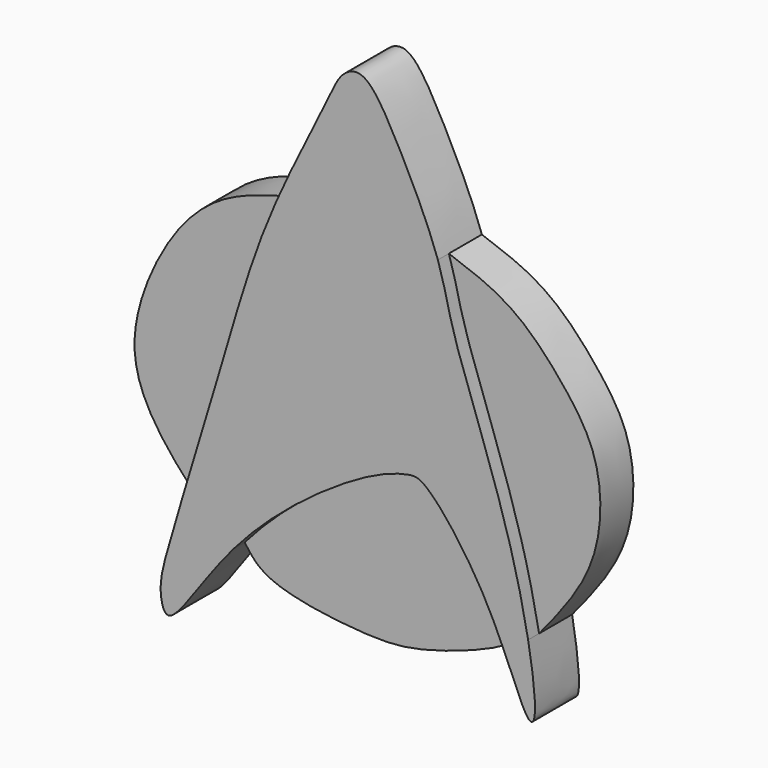
from build123d import *

# Parameters (mm, degrees)
F1_DEPTH = 10.16
F2_DEPTH = 7.62


# Not quite as in the source:
# - a feature names something its author has since deleted; it is built from what else it names


with BuildPart() as f1:
    # F0 (on Front) → F1 (new body)
    with BuildSketch(Plane.XZ):
        with BuildLine():
            add(Edge.make_bspline(
                [(28.992260687, -51.125045095), (28.3542685584, -47.6041133313), (24.5731440192, -30.3142446822), (14.6542496305, -6.5082500378), (13.6472214399, 1.3233310586), (12.3196523637, 5.2555091679)],
                knots=[0.8432322735, 0.8432322735, 0.8432322735, 0.8432322735, 0.8677839764, 0.9518885045, 1, 1, 1, 1], degree=3))
            add(Edge.make_bspline(
                [(12.3196523637, 5.2555091679), (10.61980651, 10.290348239), (4.9500571604, 22.0767618937), (-0.9757985337, 31.9404522882), (-5.7479640246, 30.0120107701), (-8.2004857079, 23.9136843789), (-14.3824154124, 12.2416093831), (-17.6358987441, 4.8334208231)],
                knots=[0, 0, 0, 0, 0.0616029159, 0.1066291224, 0.1322179197, 0.1677258873, 0.2305197427, 0.2305197427, 0.2305197427, 0.2305197427], degree=3))
            add(Edge.make_bspline(
                [(-17.6358987441, 4.8334208231), (-17.9733857287, 4.0649622317), (-22.1836405162, -5.7326263077), (-26.4141695975, -20.9824695343), (-32.763153948, -41.7024504699), (-34.8875297492, -48.7852445916)],
                knots=[0.2305197427, 0.2305197427, 0.2305197427, 0.2305197427, 0.2370334103, 0.3136224027, 0.3682900919, 0.3682900919, 0.3682900919, 0.3682900919], degree=3))
            add(Edge.make_bspline(
                [(-34.8875297492, -48.7852445916), (-35.9471827463, -52.3181901349), (-38.2300866389, -60.0434285284), (-39.3566173352, -64.8119959688), (-37.4131760235, -72.2791048189), (-31.4341899312, -61.0313718112), (-25.4187397659, -54.0002956986)],
                knots=[0.3682900919, 0.3682900919, 0.3682900919, 0.3682900919, 0.3955587045, 0.4352066461, 0.460820021, 0.5224171012, 0.5224171012, 0.5224171012, 0.5224171012], degree=3))
            add(Edge.make_bspline(
                [(-25.4187397659, -54.0002956986), (-17.5845607261, -44.8434233791), (-1.5173266758, -33.6024762984), (6.7694707164, -31.3366153102), (10.2385672181, -31.2173267791), (18.9153870863, -42.0630767436), (23.5009052342, -51.982604528), (24.3885566757, -54.0002956986)],
                knots=[0.5224171012, 0.5224171012, 0.5224171012, 0.5224171012, 0.6026376236, 0.6409454024, 0.6632093958, 0.7261128605, 0.7433427512, 0.7433427512, 0.7433427512, 0.7433427512], degree=3))
            add(Edge.make_bspline(
                [(24.3885566757, -54.0002956986), (26.5903478901, -59.0051145786), (28.6394317601, -64.5177765642), (30.7238087214, -64.1336863489), (30.1629437266, -57.5857754307), (28.992260687, -51.125045095)],
                knots=[0.7433427512, 0.7433427512, 0.7433427512, 0.7433427512, 0.7860809481, 0.7981811499, 0.8432322735, 0.8432322735, 0.8432322735, 0.8432322735], degree=3))
        make_face()
    extrude(amount=F1_DEPTH)


with BuildPart() as f2:
    # F0 (on Front) → F2 (new body)
    with BuildSketch(Plane.XZ):
        with BuildLine():
            add(Edge.make_bspline(
                [(12.3196523637, 5.2555091679), (16.3293673506, 3.8357811983), (24.4648018895, 0.9552851882), (33.8214083274, -9.3522210684), (40.7356141666, -19.286508233), (40.6472321133, -36.8598470106), (32.9719946095, -46.2663130218), (28.992260687, -51.125045095)],
                knots=[0, 0, 0, 0, 0.1881816106, 0.3818643701, 0.5635006279, 0.7744831849, 1, 1, 1, 1], degree=3))
            add(Edge.make_bspline(
                [(28.992260687, -51.125045095), (28.3542685584, -47.6041133313), (24.5731440192, -30.3142446822), (14.6542496305, -6.5082500378), (13.6472214399, 1.3233310586), (12.3196523637, 5.2555091679)],
                knots=[0.8432322735, 0.8432322735, 0.8432322735, 0.8432322735, 0.8677839764, 0.9518885045, 1, 1, 1, 1], degree=3))
        make_face()
    extrude(amount=F2_DEPTH)


with BuildPart() as f2b:
    # F0 (on Front) → F2, piece 2 (new body)
    with BuildSketch(Plane.XZ):
        with BuildLine():
            add(Edge.make_bspline(
                [(-25.4187397659, -54.0002956986), (-24.3165414563, -55.5440490563), (-21.3853374114, -59.6495317512), (-3.0994731674, -61.9540870824), (6.3787545796, -61.5581423049), (19.8107127549, -56.901060642), (23.1179069318, -54.8054468343), (24.3885566757, -54.0002956986)],
                knots=[0, 0, 0, 0, 0.1575601247, 0.4190179487, 0.6250340965, 0.8559351814, 1, 1, 1, 1], degree=3))
            add(Edge.make_bspline(
                [(-25.4187397659, -54.0002956986), (-17.5845607261, -44.8434233791), (-1.5173266758, -33.6024762984), (6.7694707164, -31.3366153102), (10.2385672181, -31.2173267791), (18.9153870863, -42.0630767436), (23.5009052342, -51.982604528), (24.3885566757, -54.0002956986)],
                knots=[0.5224171012, 0.5224171012, 0.5224171012, 0.5224171012, 0.6026376236, 0.6409454024, 0.6632093958, 0.7261128605, 0.7433427512, 0.7433427512, 0.7433427512, 0.7433427512], degree=3))
        make_face()
    extrude(amount=F2_DEPTH)


with BuildPart() as f2c:
    # F0 (on Front) → F2, piece 3 (new body)
    with BuildSketch(Plane.XZ):
        with BuildLine():
            add(Edge.make_bspline(
                [(-17.6358987441, 4.8334208231), (-17.9733857287, 4.0649622317), (-22.1836405162, -5.7326263077), (-26.4141695975, -20.9824695343), (-32.763153948, -41.7024504699), (-34.8875297492, -48.7852445916)],
                knots=[0.2305197427, 0.2305197427, 0.2305197427, 0.2305197427, 0.2370334103, 0.3136224027, 0.3682900919, 0.3682900919, 0.3682900919, 0.3682900919], degree=3))
            add(Edge.make_bspline(
                [(-34.8875297492, -48.7852445916), (-37.1597512143, -46.3154286709), (-41.8636352624, -41.1162261119), (-47.9460775261, -29.0291237763), (-41.3344862222, -10.6386963733), (-31.0370320647, 1.0641410772), (-22.053409524, 3.6380541687), (-17.6358987441, 4.8334208231)],
                knots=[0, 0, 0, 0, 0.1717500879, 0.3619580647, 0.5933974335, 0.8031046848, 1, 1, 1, 1], degree=3))
        make_face()
    extrude(amount=F2_DEPTH)


solid = Compound([f1.part, f2.part, f2b.part, f2c.part])
